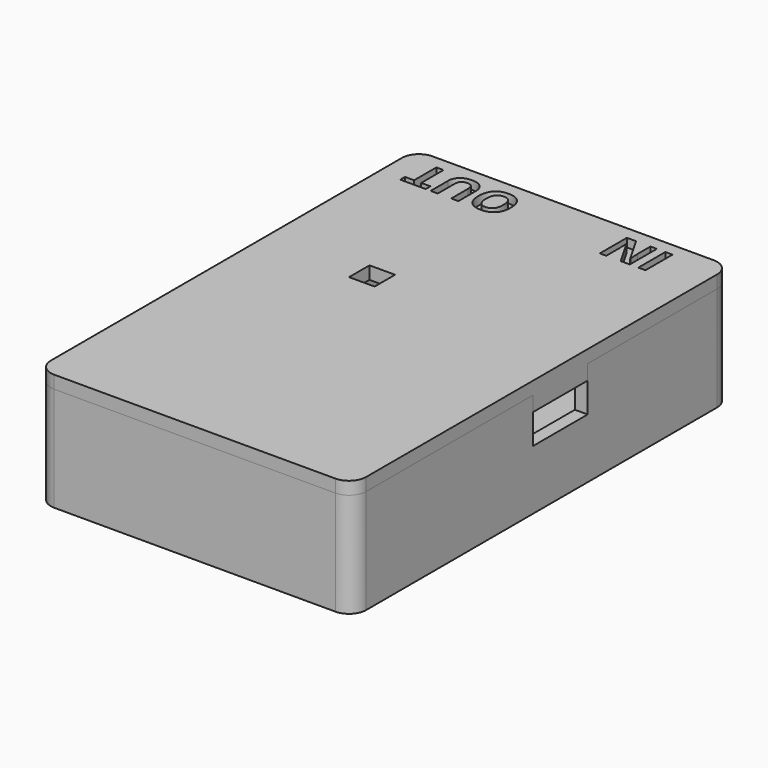
from build123d import *

# Parameters (mm, degrees)
F1_W          = 37
F1_H          = 55.5
F2_DEPTH      = 12.25
F3_T          = -1.5
F5_W          = 22
F5_H          = 12
F6_DEPTH      = 4
F7_W          = 13.5
F7_H          = 4
F8_DEPTH      = 1.5
F9_W          = 8
F9_H          = 6.5
F10_DEPTH     = 1.5
F12_DEPTH     = 1.5
F13_R         = 2
F15_DEPTH     = 7.6
F16_R         = 0.99999
F17_R         = 1
F19_DEPTH     = 1.5
F21_DEPTH     = 1.5
F23_DEPTH     = 1.5
F24_W         = 3
F24_H         = 3
F25_DEPTH     = 1.5
F26_W         = 8
F26_H         = 1.75
F27_DEPTH     = 1.5
F28_TEXT_SIZE = 5.5555555556
F29_DEPTH     = 1


# Not quite as in the source:
# - a fillet or chamfer is up to 0.001 mm smaller than in the source, because OpenCascade refuses the exact size
# - Text() gives the source's letters only with a copy of the font that has no kerning and outlines rounded to 1/6400 em; it was checked with that copy


with BuildPart() as f2:
    # F1 (on Top) → F2 (new body)
    with BuildSketch(Plane.XY):
        Rectangle(F1_W, F1_H)
    extrude(amount=F2_DEPTH)

    # F3
    f3_openings = [f2.faces().sort_by_distance(p)[0] for p in [
        (0, 0, 12.25),
    ]]
    offset(amount=F3_T, openings=f3_openings)

    # F5 (on face) → F6 (join, through all)
    with BuildSketch(Plane.XY.offset(1.5)):
        with Locations((6, -20.25)):
            Rectangle(F5_W, F5_H)
    extrude(amount=F6_DEPTH)

    # F7 (on face) → F8 (cut, through all)
    with BuildSketch(Plane(origin=(-18.5, 0, 0), x_dir=(0, -1, 0), z_dir=(-1, 0, 0))):
        with Locations((-3, 9)):
            Rectangle(F7_W, F7_H)
    extrude(amount=-F8_DEPTH, mode=Mode.SUBTRACT)

    # F9 (on face) → F10 (cut, through all)
    with BuildSketch(Plane.YZ.offset(18.5)):
        with Locations((2.75, 10.25)):
            Rectangle(F9_W, F9_H)
    extrude(amount=-F10_DEPTH, mode=Mode.SUBTRACT)

    # F11 (on face) → F12 (cut, through all)
    with BuildSketch(Plane(origin=(0, 27.75, 0), x_dir=(-1, 0, 0), z_dir=(0, 1, 0))):
        with BuildLine():
            Line((-13, 12.25), (-13, 9.5))
            ThreePointArc((-13, 9.5), (-10.25, 6.75), (-7.5, 9.5))
            Line((-7.5, 9.5), (-7.5, 12.25))
            Line((-7.5, 12.25), (-13, 12.25))
        make_face()
        with BuildLine():
            ThreePointArc((7.5, 9.5), (10.25, 6.75), (13, 9.5))
            Line((13, 9.5), (13, 12.25))
            Line((13, 12.25), (7.5, 12.25))
            Line((7.5, 12.25), (7.5, 9.5))
        make_face()
    extrude(amount=-F12_DEPTH, mode=Mode.SUBTRACT)

    # F13
    f13_edges = [f2.edges().sort_by_distance(p)[0] for p in [
        (-18.5, 27.75, 6.125),
        (18.5, 27.75, 6.125),
        (-18.5, -27.75, 6.125),
        (18.5, -27.75, 6.125),
    ]]
    fillet(f13_edges, radius=F13_R)

    # F14 (on face) → F15 (cut)
    with BuildSketch(Plane.XY.offset(12.25)):
        with BuildLine():
            ThreePointArc((-18, -17.25), (-17.7071067812, -17.9571067812), (-17, -18.25))
            Line((-17, -18.25), (-17, -9.25))
            ThreePointArc((-17, -9.25), (-17.7071067812, -9.5428932188), (-18, -10.25))
            Line((-18, -10.25), (-18, -17.25))
        make_face()
    extrude(amount=-F15_DEPTH, mode=Mode.SUBTRACT)

    # F16 (radius 1 in the source; OpenCascade refuses exactly that, so slightly less here)
    f16_edges = [f2.edges().sort_by_distance(p)[0] for p in [
        (-18, -13.75, 4.65),
    ]]
    fillet(f16_edges, radius=F16_R)

    # F17
    f17_edges = [f2.edges().sort_by_distance(p)[0] for p in [
        (-17, -17.95711, 4.94289),
        (-17, -9.54289, 4.94289),
    ]]
    fillet(f17_edges, radius=F17_R)


with BuildPart() as f19:
    # F18 (on face) → F19 (new body)
    with BuildSketch(Plane.XY.offset(12.25)):
        with BuildLine():
            Line((16.5, 27.75), (-16.5, 27.75))
            ThreePointArc((-16.5, 27.75), (-17.9142135624, 27.1642135624), (-18.5, 25.75))
            Line((-18.5, 25.75), (-18.5, -25.75))
            ThreePointArc((-18.5, -25.75), (-17.9142135624, -27.1642135624), (-16.5, -27.75))
            Line((-16.5, -27.75), (16.5, -27.75))
            ThreePointArc((16.5, -27.75), (17.9142135624, -27.1642135624), (18.5, -25.75))
            Line((18.5, -25.75), (18.5, 25.75))
            ThreePointArc((18.5, 25.75), (17.9142135624, 27.1642135624), (16.5, 27.75))
        make_face()
    extrude(amount=F19_DEPTH)

    # F20 (on face) → F21 (join, through all)
    with BuildSketch(Plane(origin=(0, 27.75, 0), x_dir=(-1, 0, 0), z_dir=(0, 1, 0))):
        with BuildLine():
            ThreePointArc((-12.3713203436, 11.25), (-11.42260394, 11.9874685928), (-10.25, 12.25))
            Line((-10.25, 12.25), (-13, 12.25))
            Line((-13, 12.25), (-13, 11.25))
            Line((-13, 11.25), (-12.3713203436, 11.25))
        make_face()
        with BuildLine():
            Line((-7.5, 11.25), (-7.5, 12.25))
            Line((-7.5, 12.25), (-10.25, 12.25))
            ThreePointArc((-10.25, 12.25), (-9.07739606, 11.9874685928), (-8.1286796564, 11.25))
            Line((-8.1286796564, 11.25), (-7.5, 11.25))
        make_face()
        with BuildLine():
            Line((10.25, 12.25), (7.5, 12.25))
            Line((7.5, 12.25), (7.5, 11.25))
            Line((7.5, 11.25), (8.1286796564, 11.25))
            ThreePointArc((8.1286796564, 11.25), (9.07739606, 11.9874685928), (10.25, 12.25))
        make_face()
        with BuildLine():
            Line((13, 12.25), (10.25, 12.25))
            ThreePointArc((10.25, 12.25), (11.42260394, 11.9874685928), (12.3713203436, 11.25))
            Line((12.3713203436, 11.25), (13, 11.25))
            Line((13, 11.25), (13, 12.25))
        make_face()
    extrude(amount=-F21_DEPTH)

    # F22 (on face) → F23 (join)
    with BuildSketch(Plane(origin=(0, 0, 12.25), x_dir=(1, 0, 0), z_dir=(0, 0, -1))):
        Polygon((14, -26.25), (17, -26.25), (17, 26.25), (-17, 26.25), (-17, -26.25), (-14, -26.25), (-14, 23.25), (14, 23.25), align=None)
    extrude(amount=F23_DEPTH)

    # F24 (on face) → F25 (cut, through all)
    with BuildSketch(Plane.XY.offset(13.75)):
        with Locations((-6, 5.75)):
            Rectangle(F24_W, F24_H)
    extrude(amount=-F25_DEPTH, mode=Mode.SUBTRACT)

    # F26 (on face) → F27 (join, through all)
    with BuildSketch(Plane.YZ.offset(17)):
        with Locations((2.75, 11.375)):
            Rectangle(F26_W, F26_H)
    extrude(amount=F27_DEPTH)

    # F28 (on face) → F29 (cut)
    with BuildSketch(Plane.XY.offset(13.75)):
        with Locations(Location((13.3585069444, 26.25), (0, 0, 180))):
            Text('IN', F28_TEXT_SIZE, font='Open Sans', font_style=FontStyle.BOLD, text_align=(TextAlign.LEFT, TextAlign.BOTTOM))
        with Locations(Location((-4.2061631944, 26.25), (0, 0, 180))):
            Text('OUT', F28_TEXT_SIZE, font='Open Sans', font_style=FontStyle.BOLD, text_align=(TextAlign.LEFT, TextAlign.BOTTOM))
    extrude(amount=-F29_DEPTH, mode=Mode.SUBTRACT)


solid = Compound([f2.part, f19.part])
